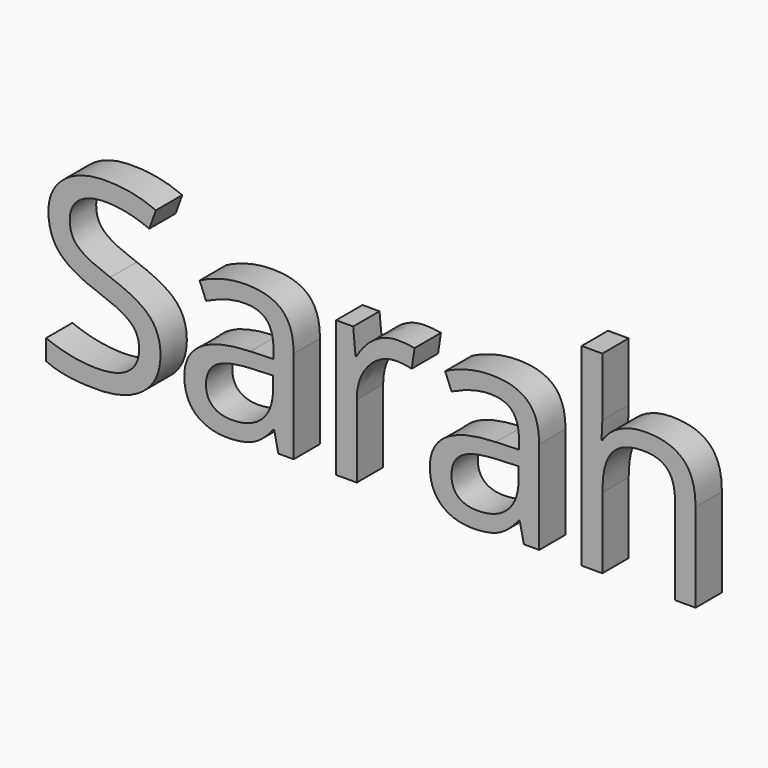
from build123d import *

# Parameters (mm, degrees)
F0_TEXT_SIZE = 49.0564697733
F1_DEPTH     = 6.35


# Not quite as in the source:
# - Text() gives the source's letters only with a copy of the font that has no kerning and outlines rounded to 1/6400 em; it was checked with that copy


with BuildPart() as f1:
    # F0 (on Front) → F1 (new body)
    with BuildSketch(Plane.XZ):
        with Locations((-69.0188258886, -16.6843924671)):
            Text('Sarah', F0_TEXT_SIZE, font='Open Sans', text_align=(TextAlign.LEFT, TextAlign.BOTTOM))
    extrude(amount=F1_DEPTH)


solid = f1.part
